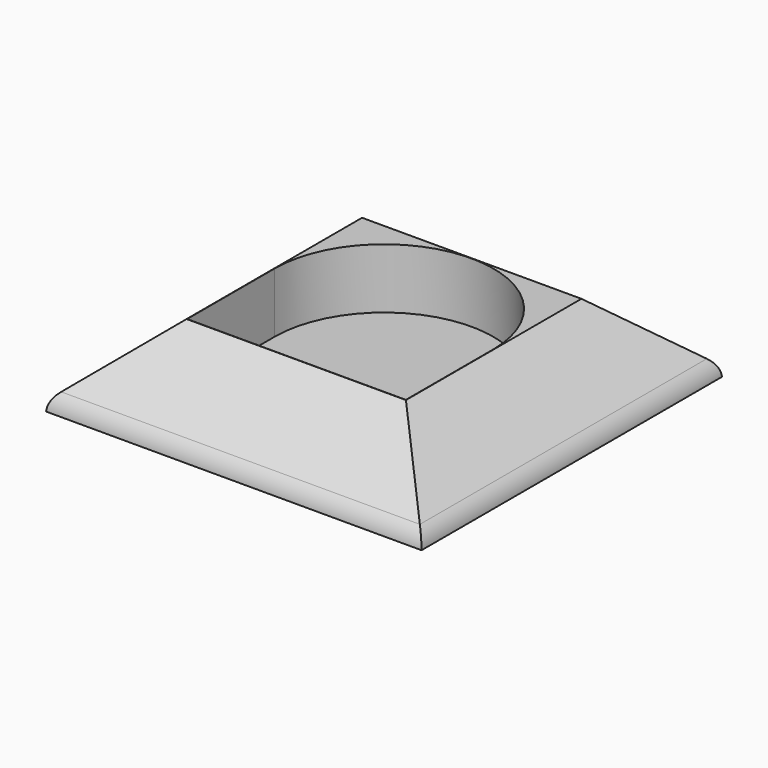
from build123d import *

# Parameters (mm, degrees)
F0_W        = 31.75
F0_H        = 31.75
F1_DEPTH    = 6.35
F2_SIZE2    = 5.5380575658
F2_SIZE     = 6.6
F4_DEPTH    = 5.08
F5_T1_DEPTH = 36.3880046162
F5_T3_DEPTH = 36.3880046162


# Not quite as in the source:
# - a fillet or chamfer that OpenCascade refuses, or shapes differently, is made with other operations: its cross-section is extruded or revolved along the edge and cut away or added


with BuildPart() as f1:
    # F0 (on Top) → F1 (new body)
    with BuildSketch(Plane.XY):
        Rectangle(F0_W, F0_H)
    extrude(amount=F1_DEPTH)

    # F2
    f2_edges = [f1.edges().sort_by_distance(p)[0] for p in [
        (-15.875, 0, 6.35),
        (0, -15.875, 6.35),
        (15.875, 0, 6.35),
        (0, 15.875, 6.35),
    ]]
    f2_side = f1.faces().sort_by_distance((0, 0, 6.35))[0]
    chamfer(f2_edges, length=F2_SIZE, length2=F2_SIZE2, reference=f2_side)

    # F3 (on face) → F4 (cut)
    with BuildSketch(Plane.XY.offset(6.35)):
        with BuildLine():
            Line((9.25, -9.25), (9.25, 0))
            ThreePointArc((9.25, 0), (0, 9.25), (-9.25, 0))
            Line((-9.25, 0), (-9.25, -9.25))
            Line((-9.25, -9.25), (9.25, -9.25))
        make_face()
    extrude(amount=-F4_DEPTH, mode=Mode.SUBTRACT)

    # F5: fillet of radius 2 on 4 edges, made by hand

    # F5_s2 → F5_t1 (cut)
    with BuildSketch(Plane.YZ.offset(-18.1940023081)):
        with BuildLine():
            ThreePointArc((-15.875, 0), (-15.6643933238, 0.7771054734), (-15.1644164673, 1.4081928144))
            Line((-15.1644164673, 1.4081928144), (-15.875, 0.8119424342))
            Line((-15.875, 0.8119424342), (-15.875, 0))
        make_face()
        with BuildLine():
            ThreePointArc((15.875, 0), (15.6643933238, 0.7771054734), (15.1644164673, 1.4081928144))
            Line((15.1644164673, 1.4081928144), (15.875, 0.8119424342))
            Line((15.875, 0.8119424342), (15.875, 0))
        make_face()
    extrude(amount=F5_T1_DEPTH, mode=Mode.SUBTRACT)

    # F5_s4 → F5_t3 (cut)
    with BuildSketch(Plane.XZ.offset(-18.1940023081)):
        with BuildLine():
            ThreePointArc((15.875, 0), (15.6643933238, 0.7771054734), (15.1644164673, 1.4081928144))
            Line((15.1644164673, 1.4081928144), (15.875, 0.8119424342))
            Line((15.875, 0.8119424342), (15.875, 0))
        make_face()
        with BuildLine():
            ThreePointArc((-15.875, 0), (-15.6643933238, 0.7771054734), (-15.1644164673, 1.4081928144))
            Line((-15.1644164673, 1.4081928144), (-15.875, 0.8119424342))
            Line((-15.875, 0.8119424342), (-15.875, 0))
        make_face()
    extrude(amount=F5_T3_DEPTH, mode=Mode.SUBTRACT)


solid = f1.part
